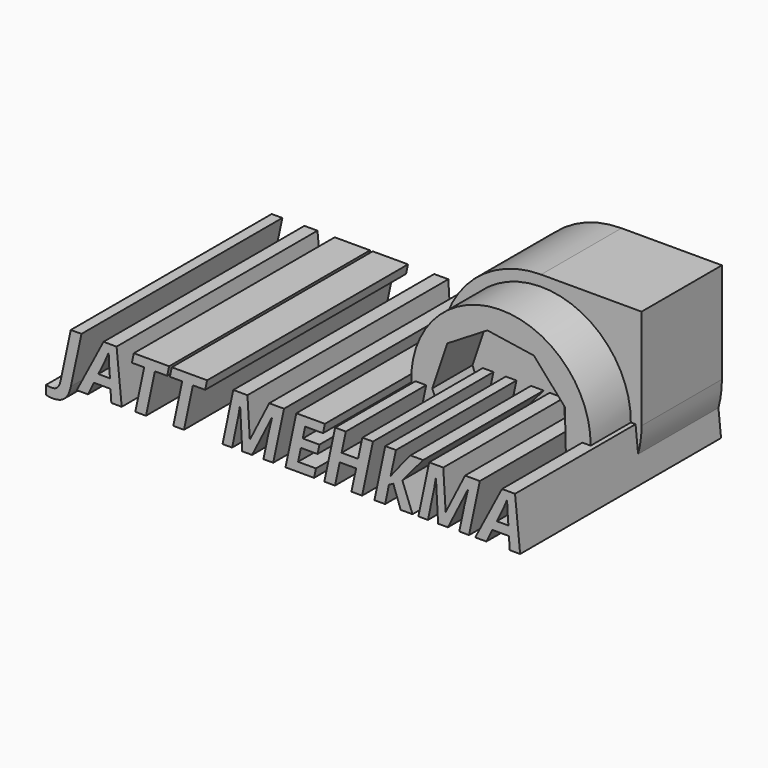
from build123d import *

# Parameters (mm, degrees)
F1_DEPTH     = 50.8
F2_R         = 45.3694407231
F3_DEPTH     = 25.4
F4_TEXT_SIZE = 36.2185218061
F5_DEPTH     = 127


# Not quite as in the source:
# - Text() gives the source's letters only with a copy of the font that has no kerning and outlines rounded to 1/6400 em; it was checked with that copy


with BuildPart() as f1:
    # F0 (on Front) → F1 (new body)
    with BuildSketch(Plane.XZ):
        with BuildLine():
            Line((-50.8, -50.8), (0, -50.8))
            ThreePointArc((0, -50.8), (35.9210244843, -35.9210244843), (50.8, 0))
            Line((50.8, 0), (50.8, 50.8))
            Line((50.8, 50.8), (0, 50.8))
            ThreePointArc((0, 50.8), (-35.9210244843, 35.9210244843), (-50.8, 0))
            Line((-50.8, 0), (-50.8, -50.8))
        make_face()
    extrude(amount=F1_DEPTH)

    # F2 (on face) → F3 (join)
    with BuildSketch(Plane.XZ.offset(50.8)):
        Circle(F2_R)
        Polygon((-34.7116861405, -0.8363516907), (-27.1282907833, 21.6715591973), (-6.8512666713, 34.0391066843), (16.6315412596, 30.4793778512), (32.3322661962, 12.658009381), (32.9043644464, -11.0861823567), (18.0801448809, -29.6430261605), (-5.2039754128, -34.3295685783), (-26.0530977751, -22.9529243276), align=None, mode=Mode.SUBTRACT)
    extrude(amount=F3_DEPTH)

    # F4 (on Front) → F5 (join)
    with BuildSketch(Plane.XZ):
        with Locations((-183.7266758084, -26.2748893583)):
            Text('JATT MEHKMA', F4_TEXT_SIZE, font='Open Sans', font_style=FontStyle.BOLDITALIC, text_align=(TextAlign.LEFT, TextAlign.BOTTOM))
    extrude(amount=F5_DEPTH)


solid = f1.part
